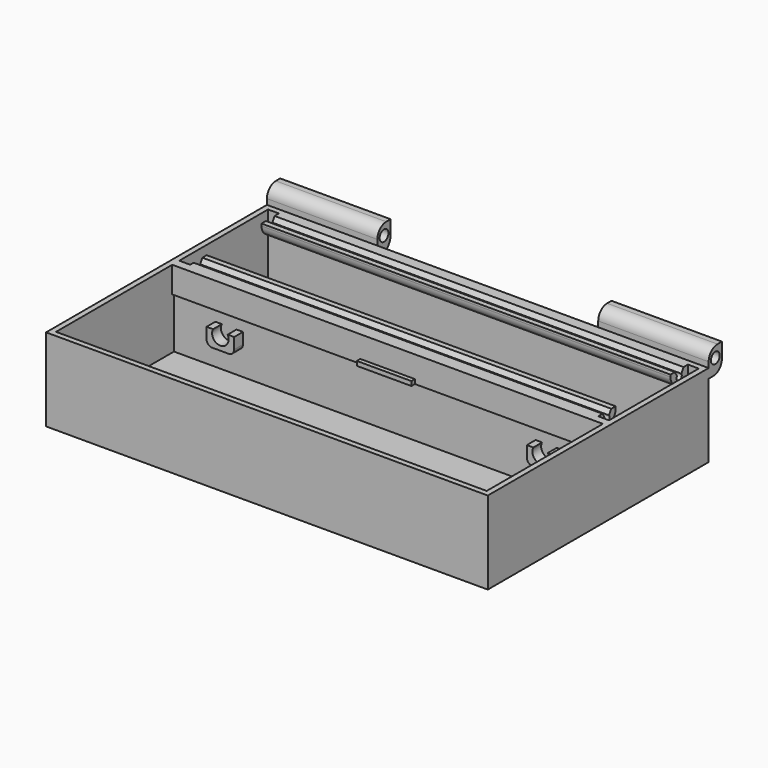
from build123d import *

# Parameters (mm, degrees)
F0_W      = 203.2
F0_H      = 127
F1_DEPTH  = 19.05
F2_T      = -2.54
F3_W      = 198.12
F3_H      = 2.54
F4_DEPTH  = 35.56
F6_DEPTH  = 5.08
F8_DEPTH  = 5.08
F9_R      = 2.54
F10_DEPTH = 50.8
F11_R     = 2.54
F12_DEPTH = 50.8
F14_DEPTH = 198.12
F15_W     = 5
F15_H     = 51.0505303715
F16_DEPTH = 10
F15_H_2   = 2.5
F15_H_3   = 5
F17_DEPTH = 25
F18_W     = 5
F18_H     = 2.5
F18_H_2   = 5
F19_DEPTH = 15
F21_DEPTH = 198.12
F22_W     = 86.5
F22_H     = 3.7755742139
F22_H_2   = 3.4886886767
F23_DEPTH = 15


with BuildPart() as f1:
    # F0 (on Top) → F1 (new body, symmetric)
    with BuildSketch(Plane.XY):
        with Locations((6.5631009638, -9.4094696285)):
            Rectangle(F0_W, F0_H)
    extrude(amount=F1_DEPTH, both=True)

    # F2
    f2_openings = [f1.faces().sort_by_distance(p)[0] for p in [
        (6.563101, -9.40947, 19.05),
    ]]
    offset(amount=F2_T, openings=f2_openings)

    # F3 (on face) → F4 (join, through all)
    with BuildSketch(Plane.XY.offset(-16.51)):
        with Locations((6.5631009638, -1.27)):
            Rectangle(F3_W, F3_H)
    extrude(amount=F4_DEPTH)

    # F5 (on face) → F6 (join)
    with BuildSketch(Plane.XZ.offset(2.54)):
        with BuildLine():
            ThreePointArc((-63.2868990362, -5.842), (-61.490847812, -5.0980512242), (-60.7468990362, -3.302))
            Line((-60.7468990362, -3.302), (-60.7468990362, 1.778))
            Line((-60.7468990362, 1.778), (-63.7272082492, 1.778))
            ThreePointArc((-63.7272082492, 1.778), (-67.0968990362, -3.81), (-70.4665898232, 1.778))
            Line((-70.4665898232, 1.778), (-73.4468990362, 1.778))
            Line((-73.4468990362, 1.778), (-73.4468990362, -3.302))
            ThreePointArc((-73.4468990362, -3.302), (-72.7029502604, -5.0980512242), (-70.9068990362, -5.842))
            Line((-70.9068990362, -5.842), (-63.2868990362, -5.842))
        make_face()
        with BuildLine():
            ThreePointArc((83.5927917508, 1.778), (80.2231009638, -3.81), (76.8534101768, 1.778))
            Line((76.8534101768, 1.778), (73.8731009638, 1.778))
            Line((73.8731009638, 1.778), (73.8731009638, -3.302))
            ThreePointArc((73.8731009638, -3.302), (74.6170497396, -5.0980512242), (76.4131009638, -5.842))
            Line((76.4131009638, -5.842), (84.0331009638, -5.842))
            ThreePointArc((84.0331009638, -5.842), (85.829152188, -5.0980512242), (86.5731009638, -3.302))
            Line((86.5731009638, -3.302), (86.5731009638, 1.778))
            Line((86.5731009638, 1.778), (83.5927917508, 1.778))
        make_face()
    extrude(amount=F6_DEPTH)

    # F7 (on face) → F8 (join)
    with BuildSketch(Plane(origin=(0, -70.3694696285, 0), x_dir=(-1, 0, 0), z_dir=(0, 1, 0))):
        with BuildLine():
            ThreePointArc((-76.8534101768, 1.778), (-80.2231009638, -3.81), (-83.5927917508, 1.778))
            Line((-83.5927917508, 1.778), (-86.5731009638, 1.778))
            Line((-86.5731009638, 1.778), (-86.5731009638, -3.302))
            ThreePointArc((-86.5731009638, -3.302), (-85.829152188, -5.0980512242), (-84.0331009638, -5.842))
            Line((-84.0331009638, -5.842), (-76.4131009638, -5.842))
            ThreePointArc((-76.4131009638, -5.842), (-74.6170497396, -5.0980512242), (-73.8731009638, -3.302))
            Line((-73.8731009638, -3.302), (-73.8731009638, 1.778))
            Line((-73.8731009638, 1.778), (-76.8534101768, 1.778))
        make_face()
        with BuildLine():
            ThreePointArc((60.7468990362, -3.302), (61.490847812, -5.0980512242), (63.2868990362, -5.842))
            Line((63.2868990362, -5.842), (70.9068990362, -5.842))
            ThreePointArc((70.9068990362, -5.842), (72.7029502604, -5.0980512242), (73.4468990362, -3.302))
            Line((73.4468990362, -3.302), (73.4468990362, 1.778))
            Line((73.4468990362, 1.778), (70.4665898232, 1.778))
            ThreePointArc((70.4665898232, 1.778), (67.0968990362, -3.81), (63.7272082492, 1.778))
            Line((63.7272082492, 1.778), (60.7468990362, 1.778))
            Line((60.7468990362, 1.778), (60.7468990362, -3.302))
        make_face()
    extrude(amount=F8_DEPTH)

    # F9 (on face) → F10 (join)
    with BuildSketch(Plane.YZ.offset(108.1631009638)):
        with BuildLine():
            Line((54.0905303715, 21.59), (54.0905303715, 14.7195085883))
            Line((54.0905303715, 14.7195085883), (56.6305303715, 14.7195085883))
            ThreePointArc((56.6305303715, 14.7195085883), (60.22263282, 16.2074061399), (61.7105303715, 19.7995085883))
            Line((61.7105303715, 19.7995085883), (61.7105303715, 26.67))
            Line((61.7105303715, 26.67), (59.1705303715, 26.67))
            ThreePointArc((59.1705303715, 26.67), (55.5784279231, 25.1821024484), (54.0905303715, 21.59))
        make_face()
        with Locations((57.9005303715, 21.59)):
            Circle(F9_R, mode=Mode.SUBTRACT)
    extrude(amount=-F10_DEPTH)

    # F11 (on face) → F12 (join)
    with BuildSketch(Plane(origin=(-95.0368990362, 0, 0), x_dir=(0, -1, 0), z_dir=(-1, 0, 0))):
        with BuildLine():
            Line((-55.3605303715, 13.97), (-54.0905303715, 13.97))
            Line((-54.0905303715, 13.97), (-54.0905303715, 19.05))
            Line((-54.0905303715, 19.05), (-54.0905303715, 21.59))
            ThreePointArc((-54.0905303715, 21.59), (-55.5784279231, 25.1821024484), (-59.1705303715, 26.67))
            Line((-59.1705303715, 26.67), (-61.7105303715, 26.67))
            Line((-61.7105303715, 26.67), (-61.7105303715, 20.32))
            ThreePointArc((-61.7105303715, 20.32), (-59.8506584321, 15.8298719395), (-55.3605303715, 13.97))
        make_face()
        with Locations((-57.9005303715, 21.59)):
            Circle(F11_R, mode=Mode.SUBTRACT)
    extrude(amount=-F12_DEPTH)

    # F13 (on face) → F14 (join, through all)
    with BuildSketch(Plane.YZ.offset(-92.4968990362)):
        with BuildLine():
            Line((46.5505303715, 13.05), (51.5505303715, 13.05))
            Line((51.5505303715, 13.05), (51.5505303715, 19.05))
            Line((51.5505303715, 19.05), (49.0505303715, 19.05))
            Line((49.0505303715, 19.05), (47.8193881256, 16.85))
            ThreePointArc((47.8193881256, 16.85), (46.5163953065, 14.5503884512), (45.3193881256, 16.906906512))
            Line((45.3193881256, 16.906906512), (44.0505303715, 19.05))
            Line((44.0505303715, 19.05), (41.5505303715, 19.05))
            Line((41.5505303715, 19.05), (41.5505303715, 18.05))
            ThreePointArc((41.5505303715, 18.05), (43.0149964656, 14.5144660941), (46.5505303715, 13.05))
        make_face()
        with BuildLine():
            Line((0, 19.05), (0, 13.05))
            Line((0, 13.05), (5, 13.05))
            ThreePointArc((5, 13.05), (8.5355339059, 14.5144660941), (10, 18.05))
            Line((10, 18.05), (10, 19.05))
            Line((10, 19.05), (7.5, 19.05))
            Line((7.5, 19.05), (6.231142246, 16.906906512))
            ThreePointArc((6.231142246, 16.906906512), (5.034135065, 14.5503884512), (3.731142246, 16.85))
            Line((3.731142246, 16.85), (2.5, 19.05))
            Line((2.5, 19.05), (0, 19.05))
        make_face()
    extrude(amount=F14_DEPTH)

    # F15 (on face) → F16 (cut)
    with BuildSketch(Plane.XY.offset(19.05)):
        with Locations((-89.9968990362, 26.0252651858)):
            Rectangle(F15_W, F15_H)
    extrude(amount=-F16_DEPTH, mode=Mode.SUBTRACT)

    # F15 (on face) → F17 (cut)
    with BuildSketch(Plane.XY.offset(19.05)):
        with Locations((-89.9968990362, 50.3005303715)):
            Rectangle(F15_W, F15_H_2)
        with Locations((-89.9968990362, 46.5505303715)):
            Rectangle(F15_W, F15_H_3)
        with Locations((-89.9968990362, 42.8005303715)):
            Rectangle(F15_W, F15_H_2)
    extrude(amount=-F17_DEPTH, mode=Mode.SUBTRACT)

    # F18 (on face) → F19 (cut)
    with BuildSketch(Plane.XY.offset(19.05)):
        with Locations((103.1231009638, 50.3005303715)):
            Rectangle(F18_W, F18_H)
        with Locations((103.1231009638, 46.5505303715)):
            Rectangle(F18_W, F18_H_2)
        with Locations((103.1231009638, 42.8005303715)):
            Rectangle(F18_W, F18_H)
        with Locations((103.1231009638, 8.75)):
            Rectangle(F18_W, F18_H)
        with Locations((103.1231009638, 5)):
            Rectangle(F18_W, F18_H_2)
        with Locations((103.1231009638, 1.25)):
            Rectangle(F18_W, F18_H)
    extrude(amount=-F19_DEPTH, mode=Mode.SUBTRACT)

    # F20 (on face) → F21 (join, through all)
    with BuildSketch(Plane.YZ.offset(-92.4968990362)):
        Polygon((-5.54, 7.05), (-2.54, 7.05), (-2.54, 19.05), (-3.54, 19.05), (-3.54, 9.05), (-5.54, 9.05), align=None)
    extrude(amount=F21_DEPTH)

    # F22 (on face) → F23 (cut)
    with BuildSketch(Plane.XY.offset(19.05)):
        with Locations((-49.2468990362, -5.4277871069)):
            Rectangle(F22_W, F22_H)
        with Locations((62.3731009638, -5.2843443383)):
            Rectangle(F22_W, F22_H_2)
    extrude(amount=-F23_DEPTH, mode=Mode.SUBTRACT)


solid = f1.part
